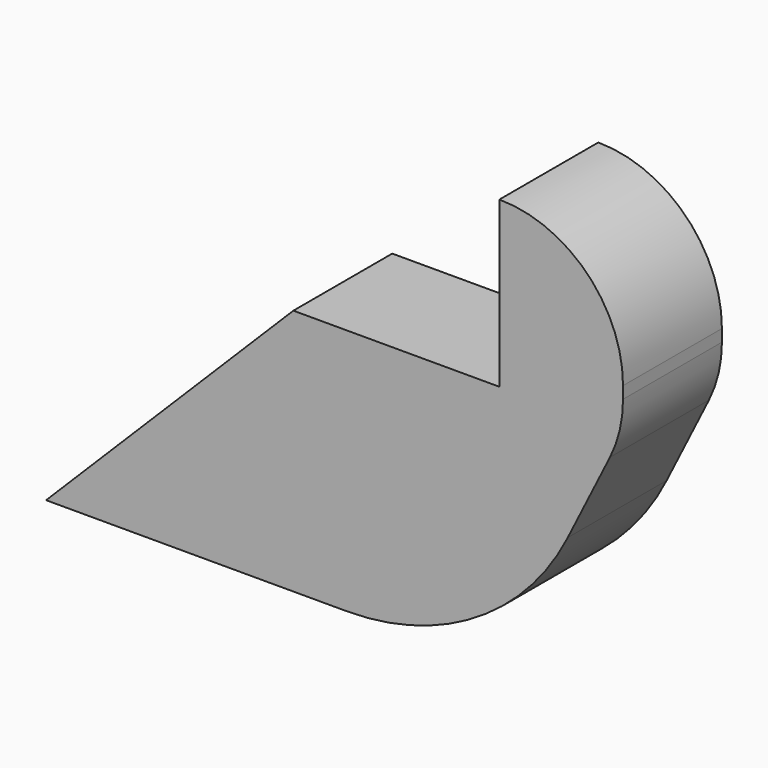
from build123d import *

# Parameters (mm, degrees)
F3_W     = 15
F3_H     = 20
F3_W_2   = 55
F3_H_2   = 30
F4_DEPTH = 15
F5_R     = 15
F6_R     = 30
F7_R     = 14.99999
F9_DEPTH = 15.001


# Not quite as in the source:
# - a fillet or chamfer is up to 0.001 mm smaller than in the source, because OpenCascade refuses the exact size


with BuildPart() as f4:
    # F3 (on Front) → F4 (new body)
    with BuildSketch(Plane.XZ):
        with Locations((7.5, 10)):
            Rectangle(F3_W, F3_H)
        with Locations((-27.5, -15)):
            Rectangle(F3_W_2, F3_H_2)
        Polygon((15, 0), (0, 0), (0, -30), align=None)
    extrude(amount=F4_DEPTH)

    # F5
    f5_edges = [f4.edges().sort_by_distance(p)[0] for p in [
        (15, -7.5, 0),
    ]]
    fillet(f5_edges, radius=F5_R)

    # F6
    f6_edges = [f4.edges().sort_by_distance(p)[0] for p in [
        (0, -7.5, -30),
    ]]
    fillet(f6_edges, radius=F6_R)

    # F7 (radius 15 in the source; OpenCascade refuses exactly that, so slightly less here)
    f7_edges = [f4.edges().sort_by_distance(p)[0] for p in [
        (15, -7.5, 20),
    ]]
    fillet(f7_edges, radius=F7_R)

    # F8 (on face) → F9 (cut, through all)
    with BuildSketch(Plane(origin=(0, 0, 0), x_dir=(-1, 0, 0), z_dir=(0, 1, 0))):
        Polygon((25, 0), (55, -30), (55, 0), align=None)
    extrude(amount=-F9_DEPTH, mode=Mode.SUBTRACT)


solid = f4.part
